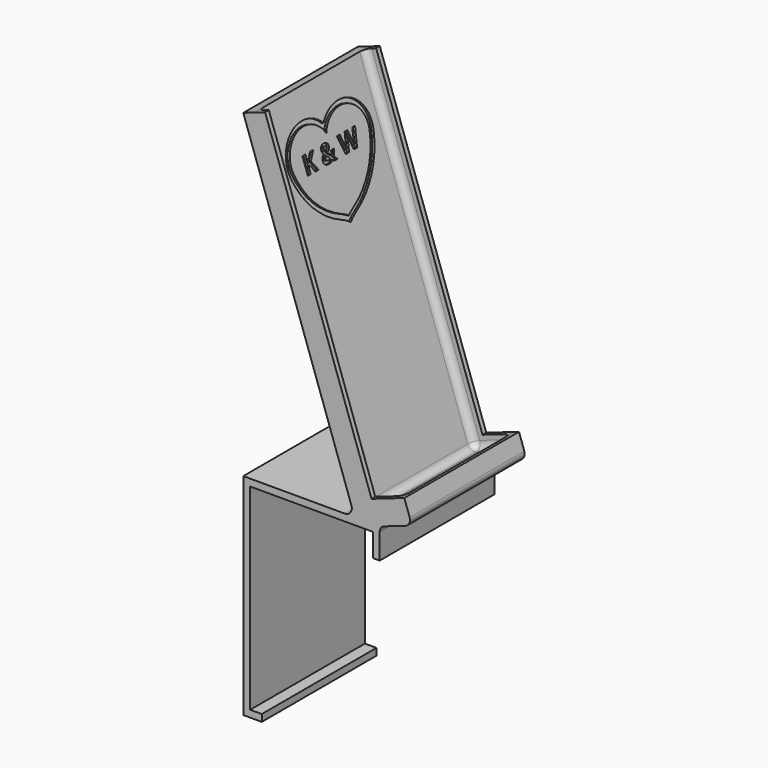
from build123d import *

# Parameters (mm, degrees)
F0_W          = 53
F0_H          = 62
F1_DEPTH      = 3
F2_W          = 3
F2_H          = 13
F3_DEPTH      = 62
F4_W          = 2
F4_H          = 145
F5_DEPTH      = 5
F6_R          = 3
F8_DEPTH      = 2
F10_DEPTH     = 2
F11_T1_DEPTH  = 52
F11_T3_DEPTH  = 2
F11_T5_DEPTH  = 12
F11_T7_DEPTH  = 2
F11_T10_ANGLE = 90
F11_T12_ANGLE = 90
F11_T14_ANGLE = 90
F11_T16_ANGLE = 90
F12_TEXT_SIZE = 10.1164444913
F13_DEPTH     = 1


# Not quite as in the source:
# - a fillet or chamfer that OpenCascade refuses, or shapes differently, is made with other operations: its cross-section is extruded or revolved along the edge and cut away or added
# - Text() gives the source's letters only with a copy of the font that has no kerning and outlines rounded to 1/6400 em; it was checked with that copy


with BuildPart() as f1:
    # F0 (on Top) → F1 (new body)
    with BuildSketch(Plane.XY):
        Rectangle(F0_W, F0_H)
    extrude(amount=F1_DEPTH)

    # F2 (on face) → F3 (join, through all)
    with BuildSketch(Plane.XZ.offset(31)):
        Polygon((-26.5, -85), (-26.5, 3), (-29.5, 3), (-29.5, -88), (-21.5, -88), (-21.5, -85), align=None)
        with Locations((28, -3.5)):
            Rectangle(F2_W, F2_H)
        Polygon((-29.5, 141.2886818262), (18.6618255138, 3), (26.5, 3), (29.5, 3), (43.4433744943, 7.8560616863), (40.1544271773, 17.2997275818), (38.2656939982, 16.6419381184), (39.9101676567, 11.9201051707), (22.9115690448, 6), (-24.7781670523, 142.9331554847), align=None)
    extrude(amount=-F3_DEPTH)

    # F4 (on face) → F5 (join)
    with BuildSketch(Plane(origin=(22.2967678276, 0, 7.7652995708), x_dir=(0, 1, 0), z_dir=(0.9443665895, 0, 0.3288947317))):
        with Locations((-30, 70.6307051834)):
            Rectangle(F4_W, F4_H)
        with Locations((30, 70.6307051834)):
            Rectangle(F4_W, F4_H)
    extrude(amount=F5_DEPTH)

    # F6
    f6_edges = [f1.edges().sort_by_distance(p)[0] for p in [
        (29.5, 0, 3),
        (43.443374, 0, 7.856062),
        (39.910168, 0, 11.920105),
        (-0.933299, 29, 74.466578),
        (-0.933299, -29, 74.466578),
        (18.661826, 0, 3),
    ]]
    fillet(f6_edges, radius=F6_R)

    # F7 (on face) → F8 (join, through all)
    with BuildSketch(Plane.XZ.offset(31)):
        with BuildLine():
            Line((25.9889283341, 12.3663066063), (27.6334019926, 7.6444736585))
            Line((27.6334019926, 7.6444736585), (37.0770678881, 10.9334209756))
            ThreePointArc((37.0770678881, 10.9334209756), (38.7913788364, 12.4609077713), (38.9234834616, 14.7532049393))
            Line((38.9234834616, 14.7532049393), (38.2656939982, 16.6419381184))
            Line((38.2656939982, 16.6419381184), (25.9889283341, 12.3663066063))
        make_face()
    extrude(amount=-F8_DEPTH)

    # F9 (on face) → F10 (join, through all)
    with BuildSketch(Plane(origin=(0, 31, 0), x_dir=(-1, 0, 0), z_dir=(0, 1, 0))):
        with BuildLine():
            Line((-37.0770678881, 10.9334209756), (-27.6334019926, 7.6444736585))
            Line((-27.6334019926, 7.6444736585), (-25.9889283341, 12.3663066063))
            Line((-25.9889283341, 12.3663066063), (-38.2656939982, 16.6419381184))
            Line((-38.2656939982, 16.6419381184), (-38.9234834616, 14.7532049393))
            ThreePointArc((-38.9234834616, 14.7532049393), (-38.7913788364, 12.4609077713), (-37.0770678881, 10.9334209756))
        make_face()
    extrude(amount=-F10_DEPTH)

    # F11: fillet of radius 3 on 9 edges, made by hand

    # F11_s2 → F11_t1 (join)
    with BuildSketch(Plane.XZ.offset(-26)):
        with BuildLine():
            ThreePointArc((21.9248848497, 8.8330997686), (23.4523716454, 7.1187888203), (25.7446688135, 6.9866841951))
            Line((25.7446688135, 6.9866841951), (22.9115690448, 6))
            Line((22.9115690448, 6), (21.9248848497, 8.8330997686))
        make_face()
    extrude(amount=F11_T1_DEPTH)

    # F11_s4 → F11_t3 (join)
    with BuildSketch(Plane(origin=(-0.3718829779, 0, 1.0678001978), x_dir=(0, 1, 0), z_dir=(-0.3288947317, 0, 0.9443665895))):
        with BuildLine():
            ThreePointArc((-29, -38.6102887103), (-28.1213203436, -40.7316090539), (-26, -41.6102887103))
            Line((-26, -41.6102887103), (-29, -41.6102887103))
            Line((-29, -41.6102887103), (-29, -38.6102887103))
        make_face()
    extrude(amount=F11_T3_DEPTH)

    # F11_s6 → F11_t5 (join)
    with BuildSketch(Plane(origin=(25.1298675963, 0, 8.7519837659), x_dir=(0, 1, 0), z_dir=(0.9443665895, 0, 0.3288947317))):
        with BuildLine():
            ThreePointArc((-29, 1.1307051834), (-28.1213203436, -0.9906151602), (-26, -1.8692948166))
            Line((-26, -1.8692948166), (-29, -1.8692948166))
            Line((-29, -1.8692948166), (-29, 1.1307051834))
        make_face()
        with BuildLine():
            ThreePointArc((29, 1.1307051834), (28.1213203436, -0.9906151602), (26, -1.8692948166))
            Line((26, -1.8692948166), (29, -1.8692948166))
            Line((29, -1.8692948166), (29, 1.1307051834))
        make_face()
    extrude(amount=F11_T5_DEPTH)

    # F11_s8 → F11_t7 (join)
    with BuildSketch(Plane(origin=(-1.0296724413, 0, 2.9565333769), x_dir=(0, 1, 0), z_dir=(0.3288947317, 0, -0.9443665895))):
        with BuildLine():
            ThreePointArc((29, 38.6102887103), (28.1213203436, 40.7316090539), (26, 41.6102887103))
            Line((26, 41.6102887103), (29, 41.6102887103))
            Line((29, 41.6102887103), (29, 38.6102887103))
        make_face()
    extrude(amount=F11_T7_DEPTH)

    # F11_s9 → F11_t10 (revolve)
    with BuildSketch(Plane(origin=(36.4622666709, 0, 12.6987205464), x_dir=(0, 1, 0), z_dir=(-0.9443665895, 0, -0.3288947317))):
        with BuildLine():
            ThreePointArc((-29, -1.1307051834), (-28.1213203436, 0.9906151602), (-26, 1.8692948166))
            Line((-26, 1.8692948166), (-29, 1.8692948166))
            Line((-29, 1.8692948166), (-29, -1.1307051834))
        make_face()
    revolve(axis=Axis((36.090383693, -29, 13.7665207442), (0, -1, 0)), revolution_arc=F11_T10_ANGLE)

    # F11_s11 → F11_t12 (revolve)
    with BuildSketch(Plane(origin=(-0.3718829779, 0, 1.0678001978), x_dir=(0, 1, 0), z_dir=(-0.3288947317, 0, 0.9443665895))):
        with BuildLine():
            ThreePointArc((26, -41.6102887103), (28.1213203436, -40.7316090539), (29, -38.6102887103))
            Line((29, -38.6102887103), (29, -41.6102887103))
            Line((29, -41.6102887103), (26, -41.6102887103))
        make_face()
    revolve(axis=Axis((36.090383693, 29, 13.7665207442), (0, 1, 0)), revolution_arc=F11_T12_ANGLE)

    # F11_s13 → F11_t14 (revolve)
    with BuildSketch(Plane.XZ.offset(-26)):
        with BuildLine():
            ThreePointArc((21.9248848497, 8.8330997686), (23.4523716454, 7.1187888203), (25.7446688135, 6.9866841951))
            Line((25.7446688135, 6.9866841951), (22.9115690448, 6))
            Line((22.9115690448, 6), (21.9248848497, 8.8330997686))
        make_face()
    revolve(axis=Axis((25.7446688135, 26, 6.9866841951), (0.3288947317, 0, -0.9443665895)), revolution_arc=F11_T14_ANGLE)

    # F11_s15 → F11_t16 (revolve)
    with BuildSketch(Plane(origin=(25.1298675963, 0, 8.7519837659), x_dir=(0, 1, 0), z_dir=(0.9443665895, 0, 0.3288947317))):
        with BuildLine():
            ThreePointArc((-26, -1.8692948166), (-28.1213203436, -0.9906151602), (-29, 1.1307051834))
            Line((-29, 1.1307051834), (-29, -1.8692948166))
            Line((-29, -1.8692948166), (-26, -1.8692948166))
        make_face()
    revolve(axis=Axis((25.7446688135, -26, 6.9866841951), (0.3288947317, 0, -0.9443665895)), revolution_arc=F11_T16_ANGLE)

    # F12 (on face) → F13 (cut)
    with BuildSketch(Plane(origin=(22.2967678276, 0, 7.7652995708), x_dir=(0, 1, 0), z_dir=(0.9443665895, 0, 0.3288947317))):
        with BuildLine():
            ThreePointArc((22.4754278478, 116.1568640653), (15.6378560582, 130.5794502977), (0, 127.3824455261))
            ThreePointArc((0, 127.3824455261), (-15.6378560582, 130.5794502977), (-22.4754278478, 116.1568640653))
            ThreePointArc((-22.4754278478, 116.1568640653), (-15.9708017214, 102.8770974157), (-4.187688546, 93.942859496))
            ThreePointArc((-4.187688546, 93.942859496), (-2.0275298394, 92.8452866441), (0, 91.51860863))
            ThreePointArc((0, 91.51860863), (2.0275298394, 92.8452866441), (4.187688546, 93.942859496))
            ThreePointArc((4.187688546, 93.942859496), (15.9708017214, 102.8770974157), (22.4754278478, 116.1568640653))
        make_face()
        with BuildLine():
            ThreePointArc((-20.5245860278, 116.5975637289), (-13.4522049285, 129.33502644), (0, 123.7404117713))
            ThreePointArc((0, 123.7404117713), (13.4522049285, 129.33502644), (20.5245860278, 116.5975637289))
            ThreePointArc((20.5245860278, 116.5975637289), (14.4267316064, 104.1482573112), (3.3804843081, 95.772728704))
            ThreePointArc((3.3804843081, 95.772728704), (1.6539423222, 94.9275813293), (0, 93.9479405232))
            ThreePointArc((0, 93.9479405232), (-1.6539423222, 94.9275813293), (-3.3804843081, 95.772728704))
            ThreePointArc((-3.3804843081, 95.772728704), (-14.4267316064, 104.1482573112), (-20.5245860278, 116.5975637289))
        make_face(mode=Mode.SUBTRACT)
        with Locations((-15, 113.6307051834)):
            Text('K & W', F12_TEXT_SIZE, font='Open Sans', font_style=FontStyle.BOLD, text_align=(TextAlign.LEFT, TextAlign.BOTTOM))
    extrude(amount=-F13_DEPTH, mode=Mode.SUBTRACT)


solid = f1.part
